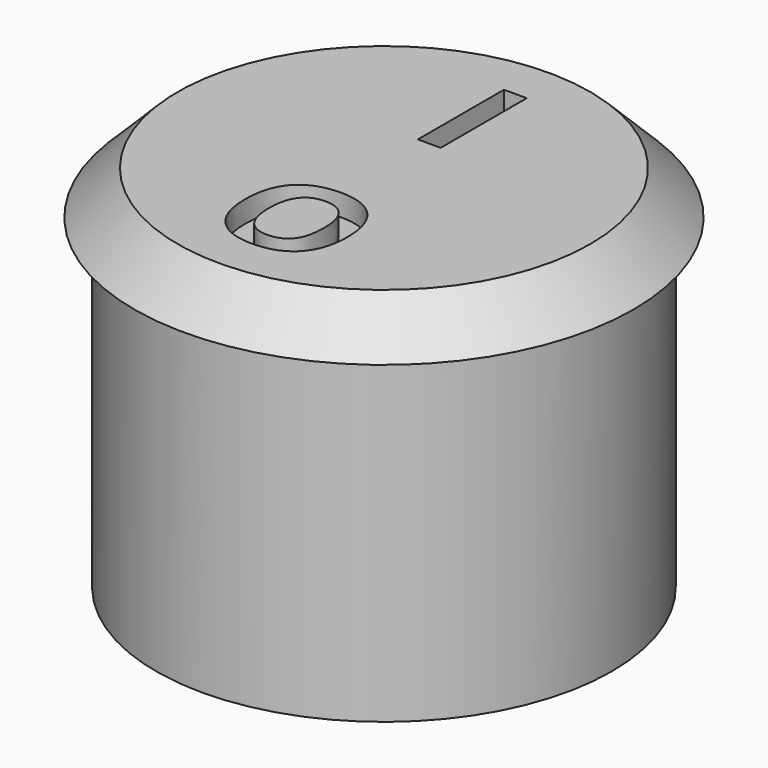
from build123d import *

# Parameters (mm, degrees)
F2_TEXT_SIZE = 6.9444444444
F3_DEPTH     = 1


# Not quite as in the source:
# - Text() gives the source's letters only with a copy of the font that has no kerning and outlines rounded to 1/6400 em; it was checked with that copy


with BuildPart() as f1:
    # F0 (on Front) → F1 (revolve)
    with BuildSketch(Plane.XZ):
        Polygon((9.5, 17), (0, 17), (0, 0), (10.5, 0), (10.5, 15), (11.5, 15), align=None)
    revolve(axis=Axis((0, 0, 8.5), (0, 0, 1)))

    # F2 (on face) → F3 (cut)
    with BuildSketch(Plane.XY.offset(17)):
        with Locations((-1.0628255208, 2.5)):
            Text('I', F2_TEXT_SIZE, font='Open Sans', font_style=FontStyle.BOLD, text_align=(TextAlign.LEFT, TextAlign.BOTTOM))
        with Locations((-2.7870008681, -7.5)):
            Text('O', F2_TEXT_SIZE, font='Open Sans', font_style=FontStyle.BOLD, text_align=(TextAlign.LEFT, TextAlign.BOTTOM))
    extrude(amount=-F3_DEPTH, mode=Mode.SUBTRACT)


solid = f1.part
